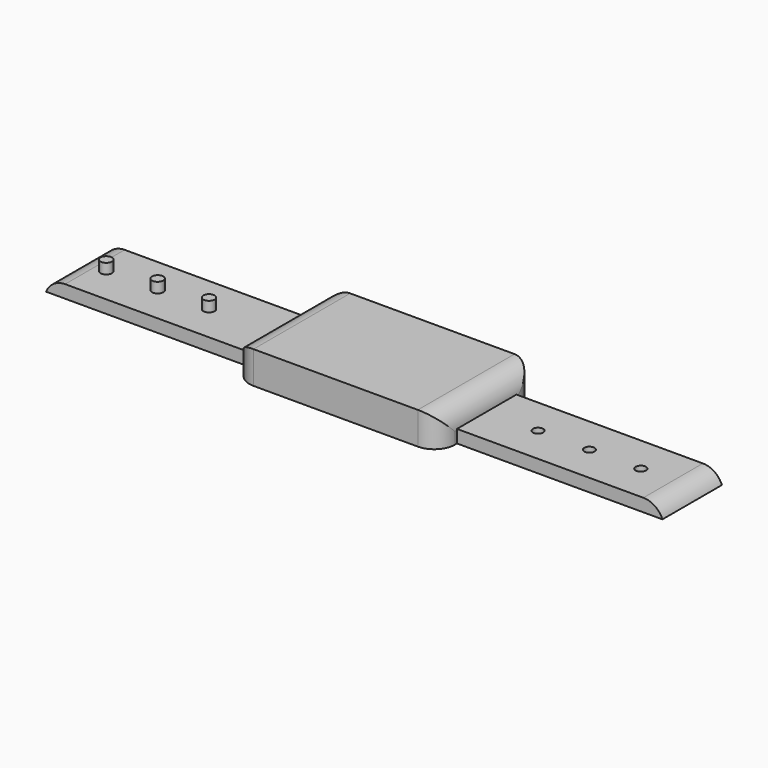
from build123d import *

# Parameters (mm, degrees)
F0_W         = 50.8
F0_H         = 18.3891410583
F1_DEPTH     = 3.175
F2_R         = 1.27
F3_DEPTH     = 25.4
F4_R         = 1.397
F5_DEPTH     = 2.54
F6_W         = 50.8
F6_H         = 29.8823560312
F7_DEPTH     = 4.826
F8_T1_DEPTH  = 33.401
F8_T6_DEPTH  = 55.2823560312
F8_T12_DEPTH = 55.2823560312
F8_T18_DEPTH = 55.2823560312
F8_T25_DEPTH = 55.2823560312
F8_T31_DEPTH = 55.2823560312
F8_T37_DEPTH = 55.2823560312
F8_T43_DEPTH = 55.2823560312
F8_T49_DEPTH = 55.2823560312
F8_T56_DEPTH = 55.2823560312
F8_T62_DEPTH = 55.2823560312
F9_T1_DEPTH  = 41.9355712549


# Not quite as in the source:
# - a fillet or chamfer that OpenCascade refuses, or shapes differently, is made with other operations: its cross-section is extruded or revolved along the edge and cut away or added


with BuildPart() as f1:
    # F0 (on Top) → F1 (new body)
    with BuildSketch(Plane.XY):
        Polygon((-25.4, -14.9411780156), (25.4, -14.9411780156), (25.4, -9.1945705292), (25.4, 9.1945705292), (25.4, 14.9411780156), (-25.4, 14.9411780156), (-25.4, 9.1945705292), (-25.4, -9.1945705292), align=None)
        with Locations((50.8, 0)):
            Rectangle(F0_W, F0_H)
        with Locations((-50.8, 0)):
            Rectangle(F0_W, F0_H)
    extrude(amount=F1_DEPTH)

    # F2 (on face) → F3 (cut)
    with BuildSketch(Plane.XY.offset(3.175)):
        with Locations((63.5, 0)):
            Circle(F2_R)
        with Locations((50.8, 0)):
            Circle(F2_R)
        with Locations((38.1, 0)):
            Circle(F2_R)
    extrude(amount=-F3_DEPTH, mode=Mode.SUBTRACT)

    # F4 (on face) → F5 (join)
    with BuildSketch(Plane.XY.offset(3.175)):
        with Locations((-68.6719441229, 0)):
            Circle(F4_R)
        with Locations((-55.9719441229, 0)):
            Circle(F4_R)
        with Locations((-43.2719441229, 0)):
            Circle(F4_R)
    extrude(amount=F5_DEPTH)

    # F6 (on face) → F7 (join)
    with BuildSketch(Plane.XY.offset(3.175)):
        Rectangle(F6_W, F6_H)
    extrude(amount=F7_DEPTH)

    # F8: fillet of radius 5.08 on 6 edges, made by hand

    # F8_s2 → F8_t1 (cut)
    with BuildSketch(Plane.XY.offset(-12.7)):
        with BuildLine():
            ThreePointArc((-20.32, 14.9411780156), (-23.9121024484, 13.453280464), (-25.4, 9.8611780156))
            Line((-25.4, 9.8611780156), (-25.4, 14.9411780156))
            Line((-25.4, 14.9411780156), (-20.32, 14.9411780156))
        make_face()
        with BuildLine():
            ThreePointArc((-20.32, -14.9411780156), (-23.9121024484, -13.453280464), (-25.4, -9.8611780156))
            Line((-25.4, -9.8611780156), (-25.4, -14.9411780156))
            Line((-25.4, -14.9411780156), (-20.32, -14.9411780156))
        make_face()
        with BuildLine():
            ThreePointArc((20.32, -14.9411780156), (23.9121024484, -13.453280464), (25.4, -9.8611780156))
            Line((25.4, -9.8611780156), (25.4, -14.9411780156))
            Line((25.4, -14.9411780156), (20.32, -14.9411780156))
        make_face()
        with BuildLine():
            ThreePointArc((20.32, 14.9411780156), (23.9121024484, 13.453280464), (25.4, 9.8611780156))
            Line((25.4, 9.8611780156), (25.4, 14.9411780156))
            Line((25.4, 14.9411780156), (20.32, 14.9411780156))
        make_face()
    extrude(amount=F8_T1_DEPTH, mode=Mode.SUBTRACT)


with BuildPart() as f8_tool4:
    # F8_s5 → F8_t6 (new body)
    with BuildSketch(Plane.XZ.offset(27.6411780156)):
        with BuildLine():
            ThreePointArc((25.4, 2.921), (23.9121024484, 6.5131024484), (20.32, 8.001))
            Line((20.32, 8.001), (25.4, 8.001))
            Line((25.4, 8.001), (25.4, 2.921))
        make_face()
    extrude(amount=-F8_T6_DEPTH)

    split(bisect_by=Plane.XY.offset(3.175), keep=Keep.BOTTOM)

    split(bisect_by=Plane.XZ.offset(9.1945705292), keep=Keep.TOP)


with BuildPart() as f1_1:
    add(f1.part)

    # F8_t3: cut F8_tool4
    add(f8_tool4.part, mode=Mode.SUBTRACT)


with BuildPart() as f8_tool10:
    # F8_s11 → F8_t12 (new body)
    with BuildSketch(Plane.XZ.offset(27.6411780156)):
        with BuildLine():
            ThreePointArc((25.4, 2.921), (23.9121024484, 6.5131024484), (20.32, 8.001))
            Line((20.32, 8.001), (25.4, 8.001))
            Line((25.4, 8.001), (25.4, 2.921))
        make_face()
    extrude(amount=-F8_T12_DEPTH)

    split(bisect_by=Plane.XY.offset(3.175), keep=Keep.TOP)

    split(bisect_by=Plane.XZ.offset(9.1945705292), keep=Keep.TOP)


with BuildPart() as f1_2:
    add(f1_1.part)

    # F8_t9: cut F8_tool10
    add(f8_tool10.part, mode=Mode.SUBTRACT)


with BuildPart() as f8_tool16:
    # F8_s17 → F8_t18 (new body)
    with BuildSketch(Plane.XZ.offset(27.6411780156)):
        with BuildLine():
            ThreePointArc((25.4, 2.921), (23.9121024484, 6.5131024484), (20.32, 8.001))
            Line((20.32, 8.001), (25.4, 8.001))
            Line((25.4, 8.001), (25.4, 2.921))
        make_face()
    extrude(amount=-F8_T18_DEPTH)

    split(bisect_by=Plane.XY.offset(3.175), keep=Keep.TOP)

    split(bisect_by=Plane.XZ.offset(-9.1945705292), keep=Keep.TOP)

    split(bisect_by=Plane.XZ.offset(9.1945705292), keep=Keep.BOTTOM)


with BuildPart() as f1_3:
    add(f1_2.part)

    # F8_t15: cut F8_tool16
    add(f8_tool16.part, mode=Mode.SUBTRACT)


with BuildPart() as f8_tool23:
    # F8_s24 → F8_t25 (new body)
    with BuildSketch(Plane.XZ.offset(27.6411780156)):
        with BuildLine():
            ThreePointArc((25.4, 2.921), (23.9121024484, 6.5131024484), (20.32, 8.001))
            Line((20.32, 8.001), (25.4, 8.001))
            Line((25.4, 8.001), (25.4, 2.921))
        make_face()
    extrude(amount=-F8_T25_DEPTH)

    split(bisect_by=Plane.XY.offset(3.175), keep=Keep.BOTTOM)

    split(bisect_by=Plane.XZ.offset(-9.1945705292), keep=Keep.BOTTOM)


with BuildPart() as f1_4:
    add(f1_3.part)

    # F8_t22: cut F8_tool23
    add(f8_tool23.part, mode=Mode.SUBTRACT)


with BuildPart() as f8_tool29:
    # F8_s30 → F8_t31 (new body)
    with BuildSketch(Plane.XZ.offset(27.6411780156)):
        with BuildLine():
            ThreePointArc((25.4, 2.921), (23.9121024484, 6.5131024484), (20.32, 8.001))
            Line((20.32, 8.001), (25.4, 8.001))
            Line((25.4, 8.001), (25.4, 2.921))
        make_face()
    extrude(amount=-F8_T31_DEPTH)

    split(bisect_by=Plane.XY.offset(3.175), keep=Keep.TOP)

    split(bisect_by=Plane.XZ.offset(-9.1945705292), keep=Keep.BOTTOM)


with BuildPart() as f1_5:
    add(f1_4.part)

    # F8_t28: cut F8_tool29
    add(f8_tool29.part, mode=Mode.SUBTRACT)


with BuildPart() as f8_tool35:
    # F8_s36 → F8_t37 (new body)
    with BuildSketch(Plane.XZ.offset(-27.6411780156)):
        with BuildLine():
            ThreePointArc((-20.32, 8.001), (-23.9121024484, 6.5131024484), (-25.4, 2.921))
            Line((-25.4, 2.921), (-25.4, 8.001))
            Line((-25.4, 8.001), (-20.32, 8.001))
        make_face()
    extrude(amount=F8_T37_DEPTH)

    split(bisect_by=Plane.XZ.offset(-9.1945705292), keep=Keep.BOTTOM)

    split(bisect_by=Plane.XY.offset(3.175), keep=Keep.TOP)


with BuildPart() as f1_6:
    add(f1_5.part)

    # F8_t34: cut F8_tool35
    add(f8_tool35.part, mode=Mode.SUBTRACT)


with BuildPart() as f8_tool41:
    # F8_s42 → F8_t43 (new body)
    with BuildSketch(Plane.XZ.offset(-27.6411780156)):
        with BuildLine():
            ThreePointArc((-20.32, 8.001), (-23.9121024484, 6.5131024484), (-25.4, 2.921))
            Line((-25.4, 2.921), (-25.4, 8.001))
            Line((-25.4, 8.001), (-20.32, 8.001))
        make_face()
    extrude(amount=F8_T43_DEPTH)

    split(bisect_by=Plane.XZ.offset(-9.1945705292), keep=Keep.BOTTOM)

    split(bisect_by=Plane.XY.offset(3.175), keep=Keep.BOTTOM)


with BuildPart() as f1_7:
    add(f1_6.part)

    # F8_t40: cut F8_tool41
    add(f8_tool41.part, mode=Mode.SUBTRACT)


with BuildPart() as f8_tool47:
    # F8_s48 → F8_t49 (new body)
    with BuildSketch(Plane.XZ.offset(-27.6411780156)):
        with BuildLine():
            ThreePointArc((-20.32, 8.001), (-23.9121024484, 6.5131024484), (-25.4, 2.921))
            Line((-25.4, 2.921), (-25.4, 8.001))
            Line((-25.4, 8.001), (-20.32, 8.001))
        make_face()
    extrude(amount=F8_T49_DEPTH)

    split(bisect_by=Plane.XZ.offset(-9.1945705292), keep=Keep.TOP)

    split(bisect_by=Plane.XY.offset(3.175), keep=Keep.TOP)

    split(bisect_by=Plane.XZ.offset(9.1945705292), keep=Keep.BOTTOM)


with BuildPart() as f1_8:
    add(f1_7.part)

    # F8_t46: cut F8_tool47
    add(f8_tool47.part, mode=Mode.SUBTRACT)


with BuildPart() as f8_tool54:
    # F8_s55 → F8_t56 (new body)
    with BuildSketch(Plane.XZ.offset(-27.6411780156)):
        with BuildLine():
            ThreePointArc((-20.32, 8.001), (-23.9121024484, 6.5131024484), (-25.4, 2.921))
            Line((-25.4, 2.921), (-25.4, 8.001))
            Line((-25.4, 8.001), (-20.32, 8.001))
        make_face()
    extrude(amount=F8_T56_DEPTH)

    split(bisect_by=Plane.XY.offset(3.175), keep=Keep.TOP)

    split(bisect_by=Plane.XZ.offset(9.1945705292), keep=Keep.TOP)


with BuildPart() as f1_9:
    add(f1_8.part)

    # F8_t53: cut F8_tool54
    add(f8_tool54.part, mode=Mode.SUBTRACT)


with BuildPart() as f8_tool60:
    # F8_s61 → F8_t62 (new body)
    with BuildSketch(Plane.XZ.offset(-27.6411780156)):
        with BuildLine():
            ThreePointArc((-20.32, 8.001), (-23.9121024484, 6.5131024484), (-25.4, 2.921))
            Line((-25.4, 2.921), (-25.4, 8.001))
            Line((-25.4, 8.001), (-20.32, 8.001))
        make_face()
    extrude(amount=F8_T62_DEPTH)

    split(bisect_by=Plane.XY.offset(3.175), keep=Keep.BOTTOM)

    split(bisect_by=Plane.XZ.offset(9.1945705292), keep=Keep.TOP)


with BuildPart() as f1_10:
    add(f1_9.part)

    # F8_t59: cut F8_tool60
    add(f8_tool60.part, mode=Mode.SUBTRACT)

    # F9: fillet of radius 5.08 on 2 edges, made by hand

    # F9_s2 → F9_t1 (cut)
    with BuildSketch(Plane.XZ.offset(-20.9677856274)):
        with BuildLine():
            ThreePointArc((71.4907139607, 3.175), (74.3305202921, 2.3071134838), (76.2, 0))
            Line((76.2, 0), (76.2, 3.175))
            Line((76.2, 3.175), (71.4907139607, 3.175))
        make_face()
        with BuildLine():
            ThreePointArc((-76.2, 0), (-74.3305202921, 2.3071134838), (-71.4907139607, 3.175))
            Line((-71.4907139607, 3.175), (-76.2, 3.175))
            Line((-76.2, 3.175), (-76.2, 0))
        make_face()
    extrude(amount=F9_T1_DEPTH, mode=Mode.SUBTRACT)


solid = f1_10.part
